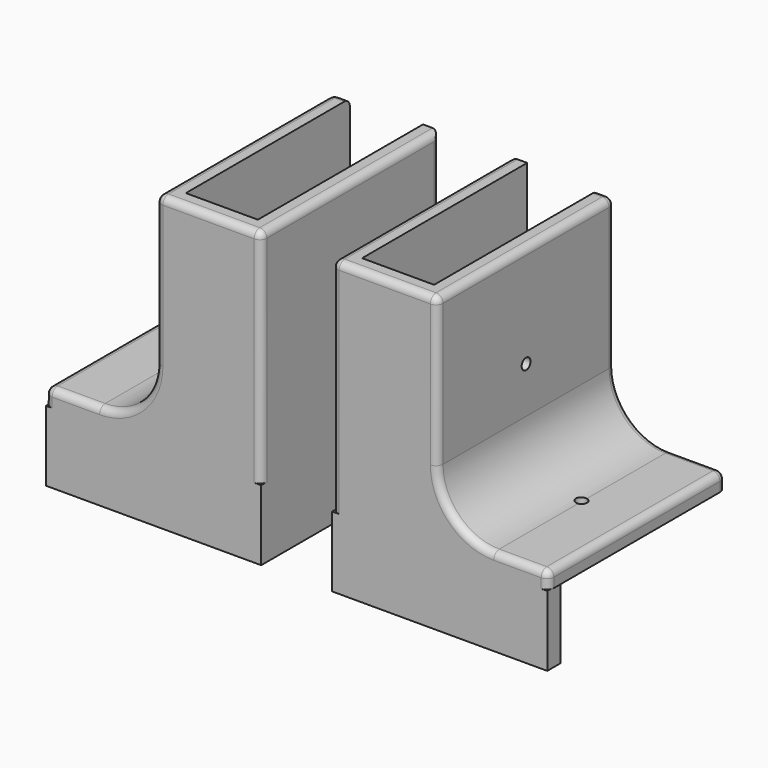
from build123d import *
from build123d import SkipClean  # not in build123d's __all__

# Parameters (mm, degrees)
F1_DEPTH     = 40
F0_W         = 20
F0_H         = 40
F0_R         = 1
F2_DEPTH     = 3
F3_R         = 1
F4_DEPTH     = 25.4
F5_R         = 1.27
F6_T4_DEPTH  = 40
F6_S5_R      = 1
F6_T6_DEPTH  = 23
F7_T1_DEPTH  = 25.57
F7_T3_DEPTH  = 8.57
F7_T5_DEPTH  = 4.905
F7_T7_DEPTH  = 4.905
F7_S11_W     = 1.27
F7_S11_H     = 1.27
F7_T12_DEPTH = 1.27
F7_T16_ANGLE = 90.0000000017
F7_T18_ANGLE = 90
F7_T20_ANGLE = 90.0000000017
F7_T22_ANGLE = 90
F7_T24_ANGLE = 90
F9_DEPTH     = 12.7
F10_DEPTH    = 22.82113
F11_R        = 1.27


# Not quite as in the source:
# - a fillet or chamfer that OpenCascade refuses, or shapes differently, is made with other operations: its cross-section is extruded or revolved along the edge and cut away or added


with BuildPart() as f1:
    # F0 (on Top) → F1 (new body)
    with BuildSketch(Plane.XY):
        Polygon((0, 40), (0, 0), (3, 0), (3, 3), (3, 40), align=None)
        Polygon((3, 3), (3, 0), (19, 0), (19, 40.2432642877), (16, 40.2432642877), (16, 3), align=None)
    extrude(amount=F1_DEPTH)

    # F0 (on Top) → F2 (join)
    with BuildSketch(Plane.XY):
        with Locations((-10, 20)):
            Rectangle(F0_W, F0_H)
        with Locations((-10, 20)):
            Circle(F0_R, mode=Mode.SUBTRACT)
        Polygon((0, 40), (0, 0), (3, 0), (3, 3), (3, 40), align=None)
        Polygon((3, 3), (3, 0), (19, 0), (19, 40.2432642877), (16, 40.2432642877), (16, 3), align=None)
    extrude(amount=F2_DEPTH)

    # F3 (on face) → F4 (cut)
    with BuildSketch(Plane(origin=(0, 0, 0), x_dir=(0, -1, 0), z_dir=(-1, 0, 0))):
        with Locations((-20, 21.5)):
            Circle(F3_R)
    extrude(amount=-F4_DEPTH, mode=Mode.SUBTRACT)

    # F5
    f5_edges = [f1.edges().sort_by_distance(p)[0] for p in [
        (-20, 20, 3),
        (0, 20, 40),
        (19, 40.243264, 20),
        (19, 20.121632, 40),
        (9.5, 0, 40),
        (19, 0, 20),
    ]]
    fillet(f5_edges, radius=F5_R)

    # F6: fillet of radius 10.16 on 1 edges, made by hand


with BuildPart() as f6_tool2:
    # F6_s3 → F6_t4 (new body)
    with BuildSketch(Plane.XZ.offset(-40)):
        with BuildLine():
            ThreePointArc((0, 13.16), (-2.9757951031, 5.9757951031), (-10.16, 3))
            Line((-10.16, 3), (0, 3))
            Line((0, 3), (0, 13.16))
        make_face()
    extrude(amount=F6_T4_DEPTH)

    # F6_s5 → F6_t6 (cut, symmetric)
    with BuildSketch(Plane.XY.offset(8.1)):
        with Locations((-10, 20)):
            Circle(F6_S5_R)
    with SkipClean():  # cleaning this boolean's faces spoils the solid; the shape is the same uncleaned
        extrude(amount=F6_T6_DEPTH, both=True, mode=Mode.SUBTRACT)


with BuildPart() as f1_1:
    add(f1.part, clean=False)

    # F6_t1: union F6_tool2
    add(f6_tool2.part)

    # F7: fillet of radius 1.27 on 2 edges, made by hand

    # F7_s2 → F7_t1 (cut)
    with BuildSketch(Plane.XY.offset(13.16)):
        with BuildLine():
            ThreePointArc((0, 38.73), (0.3719743879, 39.6280256121), (1.27, 40))
            Line((1.27, 40), (0, 40))
            Line((0, 40), (0, 38.73))
        make_face()
        with BuildLine():
            ThreePointArc((0, 1.27), (0.3719743879, 0.3719743879), (1.27, 0))
            Line((1.27, 0), (0, 0))
            Line((0, 0), (0, 1.27))
        make_face()
    extrude(amount=F7_T1_DEPTH, mode=Mode.SUBTRACT)

    # F7_s4 → F7_t3 (cut)
    with BuildSketch(Plane.YZ.offset(-18.73)):
        with BuildLine():
            ThreePointArc((1.27, 3), (0.3719743879, 2.6280256121), (0, 1.73))
            Line((0, 1.73), (0, 3))
            Line((0, 3), (1.27, 3))
        make_face()
        with BuildLine():
            ThreePointArc((38.73, 3), (39.6280256121, 2.6280256121), (40, 1.73))
            Line((40, 1.73), (40, 3))
            Line((40, 3), (38.73, 3))
        make_face()
    extrude(amount=F7_T3_DEPTH, mode=Mode.SUBTRACT)

    # F7_s6 → F7_t5 (cut)
    with BuildSketch(Plane.XY.offset(-3.175)):
        with BuildLine():
            ThreePointArc((-20, 1.27), (-19.6280256121, 0.3719743879), (-18.73, 0))
            Line((-18.73, 0), (-20, 0))
            Line((-20, 0), (-20, 1.27))
        make_face()
        with BuildLine():
            ThreePointArc((-18.73, 40), (-19.6280256121, 39.6280256121), (-20, 38.73))
            Line((-20, 38.73), (-20, 40))
            Line((-20, 40), (-18.73, 40))
        make_face()
    extrude(amount=F7_T5_DEPTH, mode=Mode.SUBTRACT)

    # F7_s8 → F7_t7 (cut)
    with BuildSketch(Plane.YZ.offset(1.27)):
        with BuildLine():
            ThreePointArc((38.73, 40), (39.6280256121, 39.6280256121), (40, 38.73))
            Line((40, 38.73), (40, 40))
            Line((40, 40), (38.73, 40))
        make_face()
    extrude(amount=F7_T7_DEPTH, mode=Mode.SUBTRACT)


with BuildPart() as f7_tool10:
    # F7_s11 → F7_t12 (new body)
    with BuildSketch(Plane.YZ.offset(1.27)):
        with Locations((0.635, 39.365)):
            Rectangle(F7_S11_W, F7_S11_H)
    extrude(amount=-F7_T12_DEPTH)

    # F7_s13 → F7_t14 (revolve, cut)
    with BuildSketch(Plane(origin=(1.27, 1.27, 38.73), x_dir=(0, 0.7071067812, -0.7071067812), z_dir=(0, 0.7071067812, 0.7071067812))):
        with BuildLine():
            ThreePointArc((0, -1.27), (1.27, 0), (0, 1.27))
            Line((0, 1.27), (0, -1.27))
        make_face()
    revolve(axis=Axis((1.27, 1.27, 38.73), (-1, 0, 0)), mode=Mode.SUBTRACT)


with BuildPart() as f1_2:
    add(f1_1.part, clean=False)

    # F7_t9: cut F7_tool10
    add(f7_tool10.part, mode=Mode.SUBTRACT)

    # F7_s15 → F7_t16 (revolve, cut)
    with BuildSketch(Plane.XY.offset(13.1599999998)):
        with BuildLine():
            ThreePointArc((0, 1.27), (0.3719743879, 0.3719743879), (1.27, 0))
            Line((1.27, 0), (0, 0))
            Line((0, 0), (0, 1.27))
        make_face()
    revolve(axis=Axis((-10.1599999998, 0, 13.1599999998), (0, 1, 0)), revolution_arc=F7_T16_ANGLE, mode=Mode.SUBTRACT)

    # F7_s17 → F7_t18 (revolve, cut)
    with BuildSketch(Plane.XY.offset(1.73)):
        with BuildLine():
            ThreePointArc((-20, 1.27), (-19.6280256121, 0.3719743879), (-18.73, 0))
            Line((-18.73, 0), (-20, 0))
            Line((-20, 0), (-20, 1.27))
        make_face()
    revolve(axis=Axis((-18.73, 0, 1.73), (0, 1, 0)), revolution_arc=F7_T18_ANGLE, mode=Mode.SUBTRACT)

    # F7_s19 → F7_t20 (revolve, cut)
    with BuildSketch(Plane.XY.offset(13.1599999998)):
        with BuildLine():
            ThreePointArc((0, 38.73), (0.3719743879, 39.6280256121), (1.27, 40))
            Line((1.27, 40), (0, 40))
            Line((0, 40), (0, 38.73))
        make_face()
    revolve(axis=Axis((-10.1599999998, 40, 13.1599999998), (0, 1, 0)), revolution_arc=F7_T20_ANGLE, mode=Mode.SUBTRACT)

    # F7_s21 → F7_t22 (revolve, cut)
    with BuildSketch(Plane.XY.offset(38.73)):
        with BuildLine():
            ThreePointArc((0, 38.73), (0.3719743879, 39.6280256121), (1.27, 40))
            Line((1.27, 40), (0, 40))
            Line((0, 40), (0, 38.73))
        make_face()
    revolve(axis=Axis((1.27, 40, 38.73), (0, 1, 0)), revolution_arc=F7_T22_ANGLE, mode=Mode.SUBTRACT)

    # F7_s23 → F7_t24 (revolve, cut)
    with BuildSketch(Plane.XY.offset(1.73)):
        with BuildLine():
            ThreePointArc((-20, 38.73), (-19.6280256121, 39.6280256121), (-18.73, 40))
            Line((-18.73, 40), (-20, 40))
            Line((-20, 40), (-20, 38.73))
        make_face()
    revolve(axis=Axis((-18.73, 40, 1.73), (0, 1, 0)), revolution_arc=F7_T24_ANGLE, mode=Mode.SUBTRACT)

    # F0 (on Top) → F9 (join)
    with BuildSketch(Plane.XY):
        Polygon((3, 3), (3, 0), (19, 0), (19, 40.2432642877), (16, 40.2432642877), (16, 3), align=None)
    extrude(amount=-F9_DEPTH)

    # F10 (add): a face of the model
    f10_faces = [f1_2.faces().sort_by_distance(p)[0] for p in [
        (3, 1.5, -6.35),
    ]]
    extrude(f10_faces, amount=F10_DEPTH)

    # F11
    f11_edges = [f1_2.edges().sort_by_distance(p)[0] for p in [
        (19, 40.243264, -6.35),
    ]]
    fillet(f11_edges, radius=F11_R)


with BuildPart() as f12_1:
    # F12: instance of F1
    add(f1_2.part.mirror(Plane.YZ.offset(25.4)), clean=False)


solid = Compound([f1_2.part, f12_1.part])
